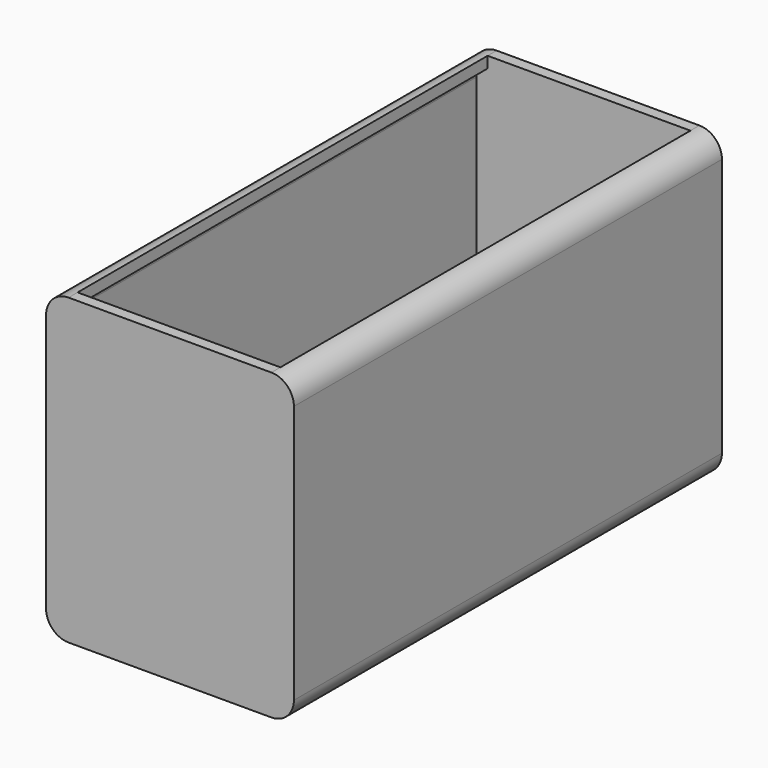
from build123d import *

# Parameters (mm, degrees)
F0_W     = 55.0703965127
F0_H     = 67.4825981259
F1_DEPTH = 118.9
F2_R     = 5
F3_T     = -2.5


# Not quite as in the source:
# - a shell that OpenCascade refuses in one call is made with other operations: the cavity is built on its own and cut out


with BuildPart() as f1:
    # F0 (on Front) → F1 (new body)
    with BuildSketch(Plane.XZ):
        Rectangle(F0_W, F0_H)
    extrude(amount=F1_DEPTH)

    # F2
    f2_edges = [f1.edges().sort_by_distance(p)[0] for p in [
        (-27.535198, -59.45, 33.741299),
        (27.535198, -59.45, 33.741299),
        (-27.535198, -59.45, -33.741299),
        (27.535198, -59.45, -33.741299),
    ]]
    fillet(f2_edges, radius=F2_R)

    # F3: a shell. OpenCascade refuses it in one call, so the cavity is built on its own and cut out:
    # the body offset inwards by the wall thickness, plus a prism from it out through each open face.
    f3_core = offset(f1.part, amount=F3_T, mode=Mode.PRIVATE)
    f3_exits = [f3_core.faces().sort_by_distance(p)[0] for p in [
        (0, -59.45, 31.241299),
    ]]
    add(f3_core, mode=Mode.SUBTRACT)
    extrude(f3_exits, amount=-F3_T, mode=Mode.SUBTRACT)


solid = f1.part
